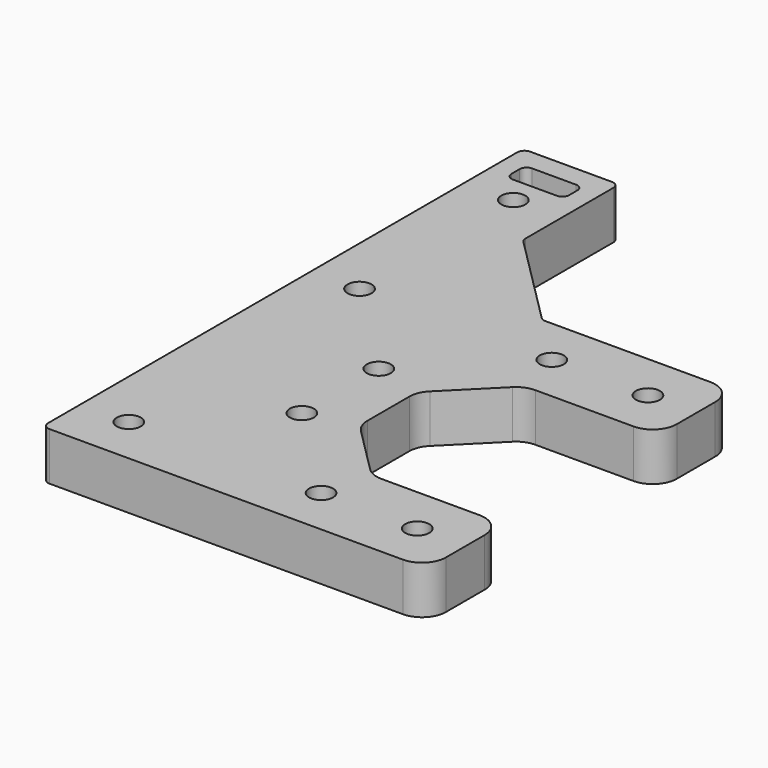
from build123d import *

# Parameters (mm, degrees)
F0_R     = 4.6
F0_R_2   = 2.5
F1_DEPTH = 10
F2_DEPTH = 7


# Not quite as in the source:
# - ends of sketch curves that miss each other by under 0.0002 mm in the source are joined


with BuildPart() as f1:
    # F0 (on Top) → F1 (new body)
    with BuildSketch(Plane.XY):
        with BuildLine():
            ThreePointArc((-40, -61), (-39.5606601718, -62.0606601718), (-38.5, -62.5))
            Line((-38.5, -62.5), (35, -62.5))
            ThreePointArc((35, -62.5), (38.5355339059, -61.0355339059), (40, -57.5))
            Line((40, -57.5), (40, -47.5))
            ThreePointArc((40, -47.5), (38.5355339059, -43.9644660941), (35, -42.5))
            Line((35, -42.5), (14.571067, -42.5))
            ThreePointArc((14.571067, -42.5), (12.6576501648, -42.1193977979), (11.0355335941, -41.0355344059))
            Line((11.0355335941, -41.0355344059), (1.464466, -31.464466))
            ThreePointArc((1.464466, -31.464466), (0.3806023374, -29.8423491618), (0, -27.928932))
            Line((0, -27.928932), (0, -17.071068))
            ThreePointArc((0, -17.071068), (0.3806023374, -15.1576508382), (1.4644660941, -13.5355340941))
            Line((1.4644660941, -13.5355340941), (11.035534, -3.964466))
            ThreePointArc((11.035534, -3.964466), (12.6576501648, -2.8806022021), (14.571067, -2.5))
            Line((14.571067, -2.5), (35, -2.5))
            ThreePointArc((35, -2.5), (38.5355339059, -1.0355339059), (40, 2.5))
            Line((40, 2.5), (40, 12.5))
            ThreePointArc((40, 12.5), (38.5355339059, 16.0355339059), (35, 17.5))
            Line((35, 17.5), (0.62132, 17.5))
            ThreePointArc((0.62132, 17.5), (0.0472948515, 17.6141807012), (-0.4393401718, 17.9393398282))
            Line((-0.4393401718, 17.9393398282), (-19.560661, 37.06066))
            ThreePointArc((-19.560661, 37.06066), (-19.8858192988, 37.5472958515), (-20, 38.121321))
            Line((-20, 38.121321), (-20, 61))
            ThreePointArc((-20, 61), (-20.4393398282, 62.0606601718), (-21.5, 62.5))
            Line((-21.5, 62.5), (-38.5, 62.5))
            ThreePointArc((-38.5, 62.5), (-39.5606601718, 62.0606601718), (-40, 61))
            Line((-40, 61), (-40, -61))
        make_face()
        with Locations((-30, -52.5)):
            Circle(F0_R, mode=Mode.SUBTRACT)
        with Locations((-10, -32.5)):
            Circle(F0_R, mode=Mode.SUBTRACT)
        with Locations((-10, -12.5)):
            Circle(F0_R, mode=Mode.SUBTRACT)
        with Locations((10, -52.5)):
            Circle(F0_R, mode=Mode.SUBTRACT)
        with Locations((30, -52.5)):
            Circle(F0_R, mode=Mode.SUBTRACT)
        with Locations((-30, 7.5)):
            Circle(F0_R, mode=Mode.SUBTRACT)
        with Locations((-30, 47.5)):
            Circle(F0_R, mode=Mode.SUBTRACT)
        with BuildLine():
            Line((-36, 54.53), (-36, 56.65))
            ThreePointArc((-36, 56.65), (-35.5782337649, 57.6682337649), (-34.56, 58.09))
            Line((-34.56, 58.09), (-25.44, 58.09))
            ThreePointArc((-25.44, 58.09), (-24.4217662351, 57.6682337649), (-24, 56.65))
            Line((-24, 56.65), (-24, 54.53))
            ThreePointArc((-24, 54.53), (-24.4217662351, 53.5117662351), (-25.44, 53.09))
            Line((-25.44, 53.09), (-34.56, 53.09))
            ThreePointArc((-34.56, 53.09), (-35.5782337649, 53.5117662351), (-36, 54.53))
        make_face(mode=Mode.SUBTRACT)
        with Locations((10, 7.5)):
            Circle(F0_R, mode=Mode.SUBTRACT)
        with Locations((30, 7.5)):
            Circle(F0_R, mode=Mode.SUBTRACT)
        with Locations((-30, 47.5)):
            Circle(F0_R)
        with Locations((-30, 47.5)):
            Circle(F0_R_2, mode=Mode.SUBTRACT)
        with Locations((-30, 7.5)):
            Circle(F0_R)
        with Locations((-30, 7.5)):
            Circle(F0_R_2, mode=Mode.SUBTRACT)
        with Locations((-30, -52.5)):
            Circle(F0_R)
        with Locations((-30, -52.5)):
            Circle(F0_R_2, mode=Mode.SUBTRACT)
        with Locations((-10, -32.5)):
            Circle(F0_R)
        with Locations((-10, -32.5)):
            Circle(F0_R_2, mode=Mode.SUBTRACT)
        with Locations((-10, -12.5)):
            Circle(F0_R)
        with Locations((-10, -12.5)):
            Circle(F0_R_2, mode=Mode.SUBTRACT)
        with Locations((10, 7.5)):
            Circle(F0_R)
        with Locations((10, 7.5)):
            Circle(F0_R_2, mode=Mode.SUBTRACT)
        with Locations((30, 7.5)):
            Circle(F0_R)
        with Locations((30, 7.5)):
            Circle(F0_R_2, mode=Mode.SUBTRACT)
        with Locations((10, -52.5)):
            Circle(F0_R)
        with Locations((10, -52.5)):
            Circle(F0_R_2, mode=Mode.SUBTRACT)
        with Locations((30, -52.5)):
            Circle(F0_R)
        with Locations((30, -52.5)):
            Circle(F0_R_2, mode=Mode.SUBTRACT)
    extrude(amount=F1_DEPTH)

    # F0 (on Top) → F2 (cut, through all)
    with BuildSketch(Plane.XY):
        with Locations((30, 7.5)):
            Circle(F0_R)
        with Locations((30, 7.5)):
            Circle(F0_R_2, mode=Mode.SUBTRACT)
        with Locations((10, 7.5)):
            Circle(F0_R)
        with Locations((10, 7.5)):
            Circle(F0_R_2, mode=Mode.SUBTRACT)
        with Locations((30, -52.5)):
            Circle(F0_R)
        with Locations((30, -52.5)):
            Circle(F0_R_2, mode=Mode.SUBTRACT)
        with Locations((10, -52.5)):
            Circle(F0_R)
        with Locations((10, -52.5)):
            Circle(F0_R_2, mode=Mode.SUBTRACT)
        with Locations((-10, -32.5)):
            Circle(F0_R)
        with Locations((-10, -32.5)):
            Circle(F0_R_2, mode=Mode.SUBTRACT)
        with Locations((-10, -12.5)):
            Circle(F0_R)
        with Locations((-10, -12.5)):
            Circle(F0_R_2, mode=Mode.SUBTRACT)
        with Locations((-30, 7.5)):
            Circle(F0_R)
        with Locations((-30, 7.5)):
            Circle(F0_R_2, mode=Mode.SUBTRACT)
        with Locations((-30, -52.5)):
            Circle(F0_R)
        with Locations((-30, -52.5)):
            Circle(F0_R_2, mode=Mode.SUBTRACT)
        with Locations((-30, 47.5)):
            Circle(F0_R)
        with Locations((-30, 47.5)):
            Circle(F0_R_2, mode=Mode.SUBTRACT)
    extrude(amount=F2_DEPTH, mode=Mode.SUBTRACT)


solid = f1.part
